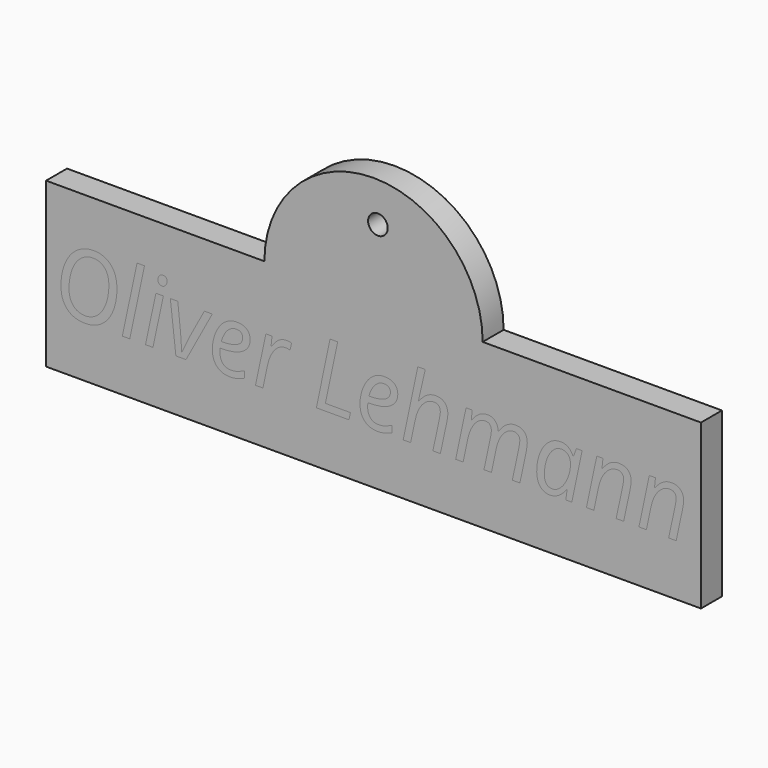
from build123d import *

# Parameters (mm, degrees)
F0_R         = 1.5
F1_DEPTH     = 4
F2_TEXT_SIZE = 13.8924942935
F3_DEPTH     = 2


# Not quite as in the source:
# - Text() gives the source's letters only with a copy of the font that has no kerning and outlines rounded to 1/6400 em; it was checked with that copy


with BuildPart() as f1:
    # F0 (on Front) → F1 (new body)
    with BuildSketch(Plane.XZ):
        Polygon((-33.333, 10.8628175019), (-33.333, -14.1371824981), (66.667, -14.1371824981), (66.667, 10.8628175019), (33.334, 10.8628175019), (0, 10.8628175019), align=None)
        with BuildLine():
            ThreePointArc((33.334, 10.8628175019), (16.667, 27.5004947461), (0, 10.8628175019))
            Line((0, 10.8628175019), (33.334, 10.8628175019))
        make_face()
        with Locations((17.3394493759, 21.4334875345)):
            Circle(F0_R, mode=Mode.SUBTRACT)
    extrude(amount=F1_DEPTH)


with BuildPart() as f3:
    # F2 (on face) → F3 (new body)
    with BuildSketch(Plane.XZ.offset(4)):
        with Locations((-32.0838354698, -6.2516223649)):
            Text('Oliver Lehmann', F2_TEXT_SIZE, font='Open Sans', font_style=FontStyle.ITALIC, text_align=(TextAlign.LEFT, TextAlign.BOTTOM))
    extrude(amount=-F3_DEPTH)


solid = Compound([f1.part, f3.part])
